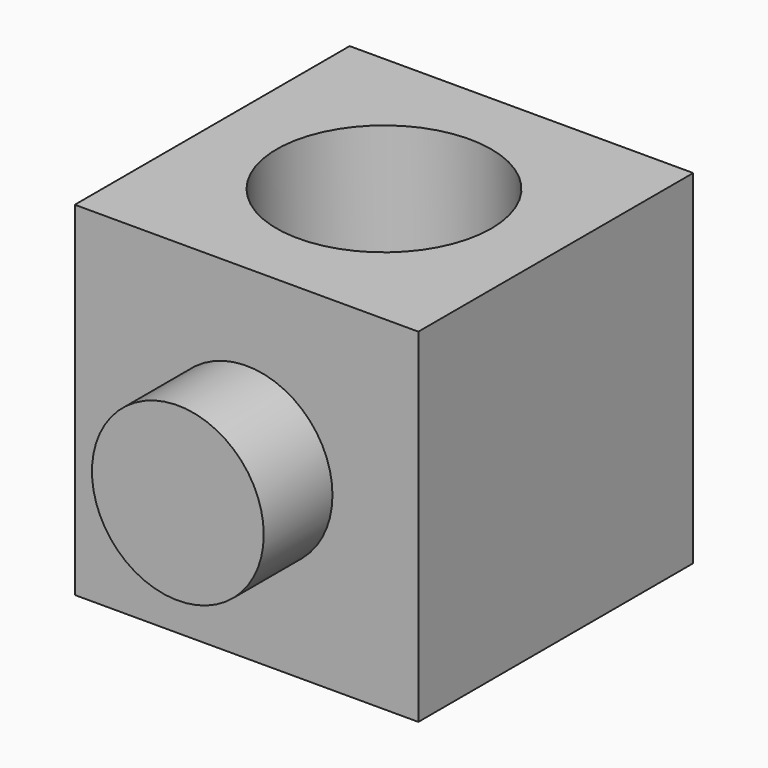
from build123d import *

# Parameters (mm, degrees)
F0_W     = 12.7
F0_H     = 12.7
F1_DEPTH = 12.7
F2_R     = 3.96875
F3_DEPTH = 12.7
F4_R     = 5.4246105656
F5_DEPTH = 6.35
F6_R     = 3.175
F7_DEPTH = 3.175


# Not quite as in the source:
# - a pattern or mirror of a feature is missing from the dataset's text; its kind, count and spacing are read off the source's solid


with BuildPart() as f1:
    # F0 (on Top) → F1 (new body)
    with BuildSketch(Plane.XY):
        Rectangle(F0_W, F0_H)
    extrude(amount=F1_DEPTH)

    # F2 (on face) → F3 (cut, through all)
    with BuildSketch(Plane.XY.offset(12.7)):
        Circle(F2_R)
    extrude(amount=-F3_DEPTH, mode=Mode.SUBTRACT)

    # F4 (on face) → F5 (cut)
    with BuildSketch(Plane(origin=(0, 0, 0), x_dir=(1, 0, 0), z_dir=(0, 0, -1))):
        Circle(F4_R)
    extrude(amount=-F5_DEPTH, mode=Mode.SUBTRACT)

    # F6 (on face) → F7 (join)
    with BuildSketch(Plane.XZ.offset(6.35)):
        with Locations((0, 6.35)):
            Circle(F6_R)
    f7 = extrude(amount=F7_DEPTH)

    # F7_copies: F7 across plane
    add(f7.mirror(Plane.ZX))


solid = f1.part
